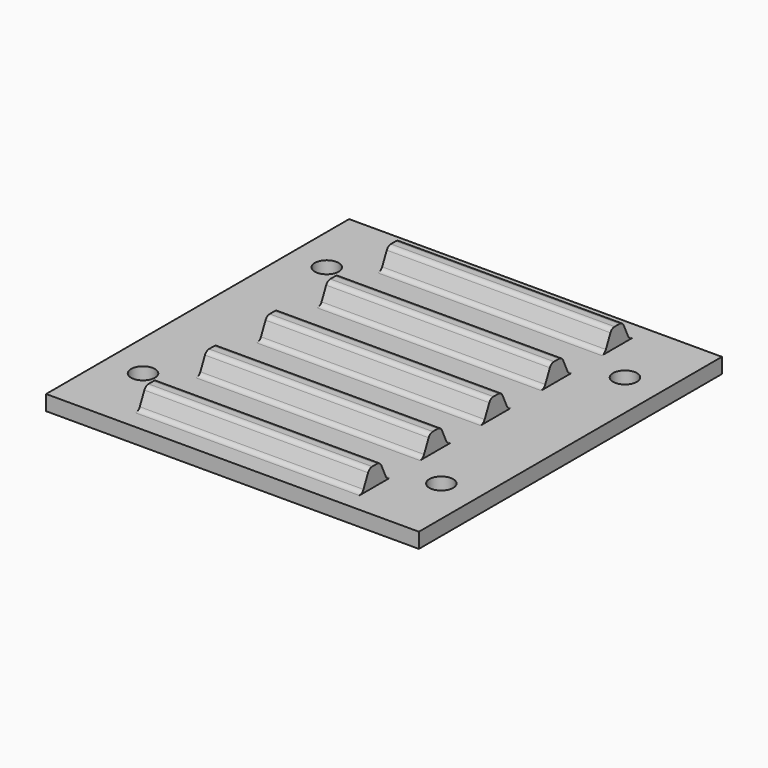
from build123d import *

# Parameters (mm, degrees)
F1_DEPTH = 7.5
F3_DEPTH = 5
F5_R     = 0.8
F6_DEPTH = 45


# Not quite as in the source:
# - ends of sketch curves that miss each other by under 0.0002 mm in the source are joined
# - a feature names something its author has since deleted; it is built from what else it names


with BuildPart() as f1:
    # F0 (on Right) → F1 (new body)
    with BuildSketch(Plane.YZ):
        with BuildLine():
            ThreePointArc((9.2226032736, 0.0929824566), (9.0820111575, -0.0673321366), (8.8773, -0.127))
            Line((8.8773, -0.127), (6.3627, -0.127))
            ThreePointArc((6.3627, -0.127), (6.1579888425, -0.0673321366), (6.0173967264, 0.0929824566))
            Line((6.0173967264, 0.0929824566), (5.6288146574, 0.9262855682))
            ThreePointArc((5.6288146574, 0.9262855682), (5.4882390894, 1.0842993961), (5.2850542, 1.143))
            Line((5.2850542, 1.143), (4.8749458, 1.143))
            ThreePointArc((4.8749458, 1.143), (4.668712979, 1.0823576494), (4.5281307776, 0.9197350317))
            Line((4.5281307776, 0.9197350317), (4.1426086033, 0.0929799713))
            ThreePointArc((4.1426086033, 0.0929799713), (4.0020111575, -0.0673321366), (3.7973, -0.127))
            Line((3.7973, -0.127), (1.2827, -0.127))
            ThreePointArc((1.2827, -0.127), (1.0779888425, -0.0673321366), (0.9373967264, 0.0929824566))
            Line((0.9373967264, 0.0929824566), (0.5488146574, 0.9262855682))
            ThreePointArc((0.5488146574, 0.9262855682), (0.4082390894, 1.0842993961), (0.2050542, 1.143))
            Line((0.2050542, 1.143), (-0.2050542, 1.143))
            ThreePointArc((-0.2050542, 1.143), (-0.411287021, 1.0823576494), (-0.5518692224, 0.9197350317))
            Line((-0.5518692224, 0.9197350317), (-0.9373913967, 0.0929799713))
            ThreePointArc((-0.9373913967, 0.0929799713), (-1.0779888425, -0.0673321366), (-1.2827, -0.127))
            Line((-1.2827, -0.127), (-3.7973, -0.127))
            ThreePointArc((-3.7973, -0.127), (-4.0020111575, -0.0673321366), (-4.1426032736, 0.0929824566))
            Line((-4.1426032736, 0.0929824566), (-4.5311853426, 0.9262855682))
            ThreePointArc((-4.5311853426, 0.9262855682), (-4.6717609106, 1.0842993961), (-4.8749458, 1.143))
            Line((-4.8749458, 1.143), (-5.2850542, 1.143))
            ThreePointArc((-5.2850542, 1.143), (-5.491287021, 1.0823576494), (-5.6318692224, 0.9197350317))
            Line((-5.6318692224, 0.9197350317), (-6.0173913967, 0.0929799713))
            ThreePointArc((-6.0173913967, 0.0929799713), (-6.1579888425, -0.0673321366), (-6.3627, -0.127))
            Line((-6.3627, -0.127), (-8.8773, -0.127))
            ThreePointArc((-8.8773, -0.127), (-9.0820111575, -0.0673321366), (-9.2226032736, 0.0929824566))
            Line((-9.2226032736, 0.0929824566), (-9.6111853426, 0.9262855682))
            ThreePointArc((-9.6111853426, 0.9262855682), (-9.7517609106, 1.0842993961), (-9.9549458, 1.143))
            Line((-9.9549458, 1.143), (-10.3650542, 1.143))
            ThreePointArc((-10.3650542, 1.143), (-10.571287021, 1.0823576494), (-10.7118692224, 0.9197350317))
            Line((-10.7118692224, 0.9197350317), (-11.0973913967, 0.0929799713))
            ThreePointArc((-11.0973913967, 0.0929799713), (-11.2379888425, -0.0673321366), (-11.4427, -0.127))
            Line((-11.4427, -0.127), (-12.7, -0.127))
            Line((-12.7, -0.127), (-12.7, -1.143))
            Line((-12.7, -1.143), (12.7, -1.143))
            Line((12.7, -1.143), (12.7, -0.127))
            Line((12.7, -0.127), (11.4427, -0.127))
            ThreePointArc((11.4427, -0.127), (11.2379888425, -0.0673321366), (11.0973967264, 0.0929824566))
            Line((11.0973967264, 0.0929824566), (10.7088146574, 0.9262855682))
            ThreePointArc((10.7088146574, 0.9262855682), (10.5682390894, 1.0842993961), (10.3650542, 1.143))
            Line((10.3650542, 1.143), (9.9549458, 1.143))
            ThreePointArc((9.9549458, 1.143), (9.748712979, 1.0823576494), (9.6081307776, 0.9197350317))
            Line((9.6081307776, 0.9197350317), (9.2226032736, 0.0929824566))
        make_face()
    extrude(amount=-F1_DEPTH)

    # F2 (on face) → F3 (join)
    with BuildSketch(Plane(origin=(-7.5, 0, 0), x_dir=(0, -1, 0), z_dir=(-1, 0, 0))):
        Polygon((-11.4427, -0.127), (-12.7, -0.127), (-12.7, -1.143), (12.7, -1.143), (12.7, -0.127), (11.4427, -0.127), (8.8773, -0.127), (6.3627, -0.127), (3.7973, -0.127), (1.2827, -0.127), (-1.2827, -0.127), (-3.7973, -0.127), (-6.3627, -0.127), (-8.8773, -0.127), align=None)
    extrude(amount=F3_DEPTH)

    # F4: F1 across plane


with BuildPart() as f1_1:
    add(f1.part)
    add(f1.part.mirror(Plane.YZ))

    # F5 (on face) → F6 (cut)
    with BuildSketch(Plane.XY.offset(-0.127)):
        with Locations((10, 7.7)):
            Circle(F5_R)
        with Locations((10, -7.7)):
            Circle(F5_R)
        with Locations((-10, 7.7)):
            Circle(F5_R)
        with Locations((-10, -7.7)):
            Circle(F5_R)
    extrude(amount=-F6_DEPTH, mode=Mode.SUBTRACT)


solid = f1_1.part
